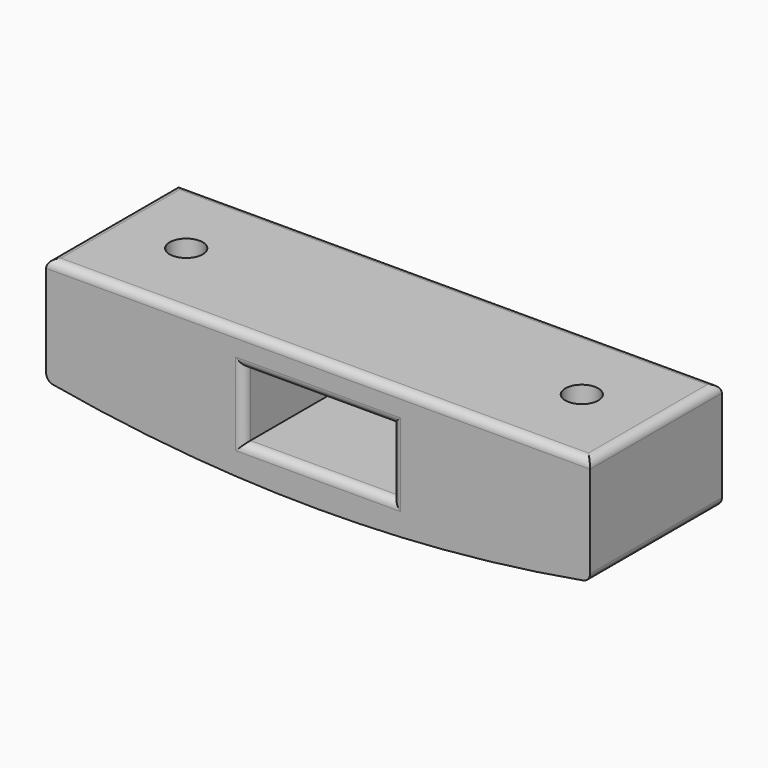
from build123d import *

# Parameters (mm, degrees)
F0_W     = 9
F0_H     = 4
F0_H_2   = 6.5
F1_DEPTH = 10
F2_R     = 0.5
F3_R     = 1
F4_DEPTH = 25


with BuildPart() as f1:
    # F0 (on Front) → F1 (new body)
    with BuildSketch(Plane.XZ):
        with BuildLine():
            ThreePointArc((-7.5, -3.6921049214), (-3.753158649, -3.9229938263), (0, -4))
            Line((0, -4), (0, -2.5))
            Line((0, -2.5), (-7.5, -2.5))
            Line((-7.5, -2.5), (-7.5, -3.6921049214))
        make_face()
        with BuildLine():
            Line((0, -2.5), (0, -4))
            ThreePointArc((0, -4), (3.753158649, -3.9229938263), (7.5, -3.6921049214))
            Line((7.5, -3.6921049214), (7.5, -2.5))
            Line((7.5, -2.5), (0, -2.5))
        make_face()
        with BuildLine():
            Line((7.5, -2.5), (7.5, -3.6921049214))
            ThreePointArc((7.5, -3.6921049214), (12.0147941529, -3.2077434482), (16.5, -2.5))
            Line((16.5, -2.5), (7.5, -2.5))
        make_face()
        Polygon((-7.5, -2.5), (0, -2.5), (7.5, -2.5), (7.5, 4), (-7.5, 4), align=None)
        Rectangle(F0_W, F0_H, mode=Mode.SUBTRACT)
        with BuildLine():
            ThreePointArc((-16.5, -2.5), (-12.0147941529, -3.2077434482), (-7.5, -3.6921049214))
            Line((-7.5, -3.6921049214), (-7.5, -2.5))
            Line((-7.5, -2.5), (-16.5, -2.5))
        make_face()
        with Locations((12, 0.75)):
            Rectangle(F0_W, F0_H_2)
        with Locations((-12, 0.75)):
            Rectangle(F0_W, F0_H_2)
    extrude(amount=F1_DEPTH)

    # F2 (call 1 of 5: OpenCascade refuses the feature's edges together)
    f2_edges = [f1.edges().sort_by_distance(p)[0] for p in [
        (16.5, -5, 4),
        (-16.5, -5, 4),
        (0, -10, 4),
        (0, 0, 4),
    ]]
    fillet(f2_edges, radius=F2_R)

    # F2#2 (call 2 of 5)
    f2_2_edges = [f1.edges().sort_by_distance(p)[0] for p in [
        (16.5, -5, -2.5),
    ]]
    fillet(f2_2_edges, radius=F2_R)

    # F2#3 (call 3 of 5)
    f2_3_edges = [f1.edges().sort_by_distance(p)[0] for p in [
        (-16.5, -5, -2.5),
    ]]
    fillet(f2_3_edges, radius=F2_R)

    # F2#4 (call 4 of 5)
    f2_4_edges = [f1.edges().sort_by_distance(p)[0] for p in [
        (-4.5, 0, 0),
        (0, 0, 2),
        (4.5, 0, 0),
        (0, 0, -2),
    ]]
    fillet(f2_4_edges, radius=F2_R)

    # F2#5 (call 5 of 5)
    f2_5_edges = [f1.edges().sort_by_distance(p)[0] for p in [
        (-4.5, -10, 0),
        (0, -10, 2),
        (4.5, -10, 0),
        (0, -10, -2),
    ]]
    fillet(f2_5_edges, radius=F2_R)

    # F3 (on face) → F4 (cut)
    with BuildSketch(Plane.XY.offset(4)):
        with Locations((-12, -5)):
            Circle(F3_R)
        with Locations((12, -5)):
            Circle(F3_R)
    extrude(amount=-F4_DEPTH, mode=Mode.SUBTRACT)


solid = f1.part
